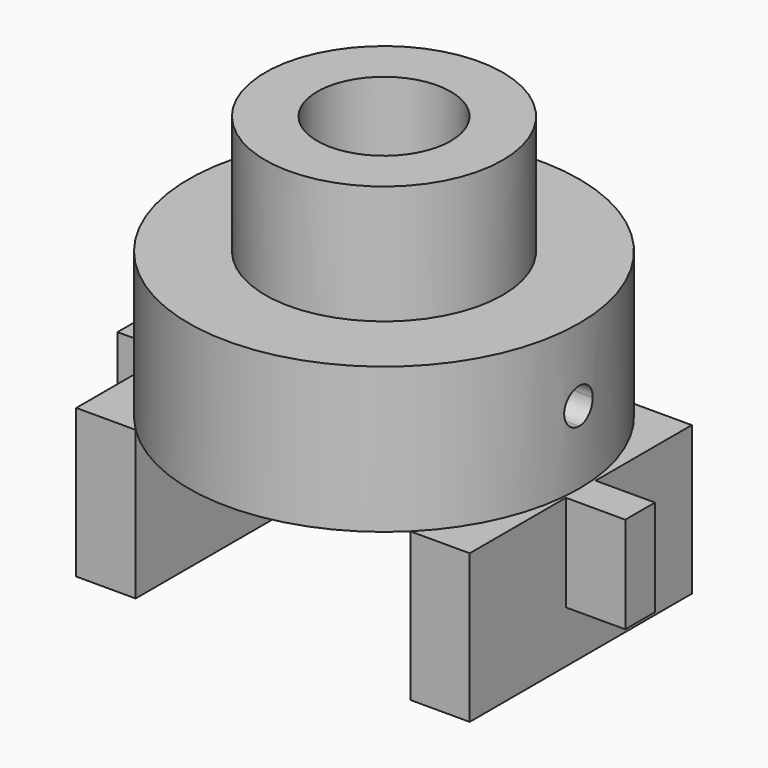
from build123d import *

# Parameters (mm, degrees)
F0_R      = 8
F0_R_2    = 4.5
F1_DEPTH  = 8
F2_R      = 13.15
F3_DEPTH  = 9.8
F4_START  = -2.8
F4_DEPTH  = 22.2
F6_DEPTH  = 10
F8_START  = -26.2
F8_DEPTH  = 4
F9_DEPTH  = 4
F10_DEPTH = 76


with BuildPart() as f1:
    # F0 (on Top) → F1 (new body)
    with BuildSketch(Plane.XY):
        Circle(F0_R)
        Circle(F0_R_2, mode=Mode.SUBTRACT)
    extrude(amount=F1_DEPTH)

    # F2 (on Top) → F3 (join)
    with BuildSketch(Plane.XY):
        Circle(F2_R)
        with BuildLine():
            ThreePointArc((-6.5986267511, 0.825), (0, 6.65), (6.5986267511, 0.825))
            Line((6.5986267511, 0.825), (6.65, 0.825))
            Line((6.65, 0.825), (9.25, 0.825))
            Line((9.25, 0.825), (9.25, -0.825))
            Line((9.25, -0.825), (6.65, -0.825))
            Line((6.65, -0.825), (6.5986267511, -0.825))
            ThreePointArc((6.5986267511, -0.825), (4.7022600949, -4.7022600949), (0.825, -6.5986267511))
            Line((0.825, -6.5986267511), (0.825, -6.65))
            Line((0.825, -6.65), (0.825, -8.25))
            Line((0.825, -8.25), (-0.825, -8.25))
            Line((-0.825, -8.25), (-0.825, -6.65))
            Line((-0.825, -6.65), (-0.825, -6.5986267511))
            ThreePointArc((-0.825, -6.5986267511), (-4.7022600949, -4.7022600949), (-6.5986267511, -0.825))
            Line((-6.5986267511, -0.825), (-6.65, -0.825))
            Line((-6.65, -0.825), (-9.25, -0.825))
            Line((-9.25, -0.825), (-9.25, 0.825))
            Line((-9.25, 0.825), (-6.65, 0.825))
            Line((-6.65, 0.825), (-6.5986267511, 0.825))
        make_face(mode=Mode.SUBTRACT)
        Polygon((-6.65, -0.825), (-6.65, 0), (-6.65, 0.825), (-9.25, 0.825), (-9.25, -0.825), align=None)
        Polygon((6.65, 0.825), (6.65, 0), (6.65, -0.825), (9.25, -0.825), (9.25, 0.825), align=None)
        Polygon((0.825, -6.65), (0, -6.65), (-0.825, -6.65), (-0.825, -8.25), (0.825, -8.25), align=None)
        with BuildLine():
            Line((0.825, -6.65), (0.825, -6.5986267511))
            ThreePointArc((0.825, -6.5986267511), (0.413298987, -6.6371442615), (0, -6.65))
            Line((0, -6.65), (0.825, -6.65))
        make_face()
        with BuildLine():
            Line((-0.825, -6.65), (0, -6.65))
            ThreePointArc((0, -6.65), (-0.413298987, -6.6371442615), (-0.825, -6.5986267511))
            Line((-0.825, -6.5986267511), (-0.825, -6.65))
        make_face()
        with BuildLine():
            ThreePointArc((6.5986267511, 0.825), (6.6371442615, 0.413298987), (6.65, 0))
            Line((6.65, 0), (6.65, 0.825))
            Line((6.65, 0.825), (6.5986267511, 0.825))
        make_face()
        with BuildLine():
            Line((6.65, -0.825), (6.65, 0))
            ThreePointArc((6.65, 0), (6.6371442615, -0.413298987), (6.5986267511, -0.825))
            Line((6.5986267511, -0.825), (6.65, -0.825))
        make_face()
        with BuildLine():
            ThreePointArc((-6.5986267511, -0.825), (-6.6371442615, -0.413298987), (-6.65, 0))
            Line((-6.65, 0), (-6.65, -0.825))
            Line((-6.65, -0.825), (-6.5986267511, -0.825))
        make_face()
        with BuildLine():
            ThreePointArc((-6.65, 0), (-6.6371442615, 0.413298987), (-6.5986267511, 0.825))
            Line((-6.5986267511, 0.825), (-6.65, 0.825))
            Line((-6.65, 0.825), (-6.65, 0))
        make_face()
    extrude(amount=-F3_DEPTH)

    # F2 (on Top) → F4 (cut)
    with BuildSketch(Plane.XY.offset(F4_START)):
        Polygon((6.65, 0.825), (6.65, 0), (6.65, -0.825), (9.25, -0.825), (9.25, 0.825), align=None)
        Polygon((0.825, -6.65), (0, -6.65), (-0.825, -6.65), (-0.825, -8.25), (0.825, -8.25), align=None)
        Polygon((-6.65, -0.825), (-6.65, 0), (-6.65, 0.825), (-9.25, 0.825), (-9.25, -0.825), align=None)
        with BuildLine():
            Line((6.65, -0.825), (6.65, 0))
            ThreePointArc((6.65, 0), (6.6371442615, -0.413298987), (6.5986267511, -0.825))
            Line((6.5986267511, -0.825), (6.65, -0.825))
        make_face()
        with BuildLine():
            ThreePointArc((6.5986267511, 0.825), (6.6371442615, 0.413298987), (6.65, 0))
            Line((6.65, 0), (6.65, 0.825))
            Line((6.65, 0.825), (6.5986267511, 0.825))
        make_face()
        with BuildLine():
            Line((-0.825, -6.65), (0, -6.65))
            ThreePointArc((0, -6.65), (-0.413298987, -6.6371442615), (-0.825, -6.5986267511))
            Line((-0.825, -6.5986267511), (-0.825, -6.65))
        make_face()
        with BuildLine():
            Line((0.825, -6.65), (0.825, -6.5986267511))
            ThreePointArc((0.825, -6.5986267511), (0.413298987, -6.6371442615), (0, -6.65))
            Line((0, -6.65), (0.825, -6.65))
        make_face()
        with BuildLine():
            ThreePointArc((-6.65, 0), (-6.6371442615, 0.413298987), (-6.5986267511, 0.825))
            Line((-6.5986267511, 0.825), (-6.65, 0.825))
            Line((-6.65, 0.825), (-6.65, 0))
        make_face()
        with BuildLine():
            ThreePointArc((-6.5986267511, -0.825), (-6.6371442615, -0.413298987), (-6.65, 0))
            Line((-6.65, 0), (-6.65, -0.825))
            Line((-6.65, -0.825), (-6.5986267511, -0.825))
        make_face()
    extrude(amount=-F4_DEPTH, mode=Mode.SUBTRACT)

    # F5 (on face) → F6 (join)
    with BuildSketch(Plane(origin=(0, 0, -9.8), x_dir=(1, 0, 0), z_dir=(0, 0, -1))):
        with BuildLine():
            ThreePointArc((13.15, 0), (12.135897165, -5.0638424146), (9.25, -9.3466571564))
            Line((9.25, -9.3466571564), (13.25, -9.3466571564))
            Line((13.25, -9.3466571564), (13.25, 9.3466571564))
            Line((13.25, 9.3466571564), (9.25, 9.3466571564))
            ThreePointArc((9.25, 9.3466571564), (12.135897165, 5.0638424146), (13.15, 0))
        make_face()
        with BuildLine():
            Line((9.25, -0.825), (9.25, -9.3466571564))
            ThreePointArc((9.25, -9.3466571564), (12.135897165, -5.0638424146), (13.15, 0))
            ThreePointArc((13.15, 0), (12.135897165, 5.0638424146), (9.25, 9.3466571564))
            Line((9.25, 9.3466571564), (9.25, 0.825))
            Line((9.25, 0.825), (9.25, -0.825))
        make_face()
        with BuildLine():
            ThreePointArc((-9.25, 9.3466571564), (-13.15, 0), (-9.25, -9.3466571564))
            Line((-9.25, -9.3466571564), (-9.25, -0.825))
            Line((-9.25, -0.825), (-9.25, 0.825))
            Line((-9.25, 0.825), (-9.25, 9.3466571564))
        make_face()
        with BuildLine():
            Line((-13.25, -9.3466571564), (-9.25, -9.3466571564))
            ThreePointArc((-9.25, -9.3466571564), (-13.15, 0), (-9.25, 9.3466571564))
            Line((-9.25, 9.3466571564), (-13.25, 9.3466571564))
            Line((-13.25, 9.3466571564), (-13.25, -9.3466571564))
        make_face()
    extrude(amount=F6_DEPTH)

    # F7 (on face) → F8 (join)
    with BuildSketch(Plane.YZ.offset(13.25).offset(F8_START)):
        Polygon((0, -9.8), (-1.25, -9.8), (-1.25, -16.3), (1.25, -16.3), (1.25, -9.8), align=None)
    extrude(amount=-F8_DEPTH)

    # F7 (on face) → F9 (join)
    with BuildSketch(Plane.YZ.offset(13.25)):
        Polygon((0, -9.8), (-1.25, -9.8), (-1.25, -16.3), (1.25, -16.3), (1.25, -9.8), align=None)
    extrude(amount=F9_DEPTH)

    # F7 (on face) → F10 (cut)
    with BuildSketch(Plane.YZ.offset(13.25)):
        with BuildLine():
            ThreePointArc((0, -3.7), (-1.2, -4.9), (0, -6.1))
            Line((0, -6.1), (0, -3.7))
        make_face()
        with BuildLine():
            Line((0, -3.7), (0, -6.1))
            ThreePointArc((0, -6.1), (0.8485281374, -5.7485281374), (1.2, -4.9))
            ThreePointArc((1.2, -4.9), (0.8485281374, -4.0514718626), (0, -3.7))
        make_face()
    extrude(amount=-F10_DEPTH, mode=Mode.SUBTRACT)


solid = f1.part
